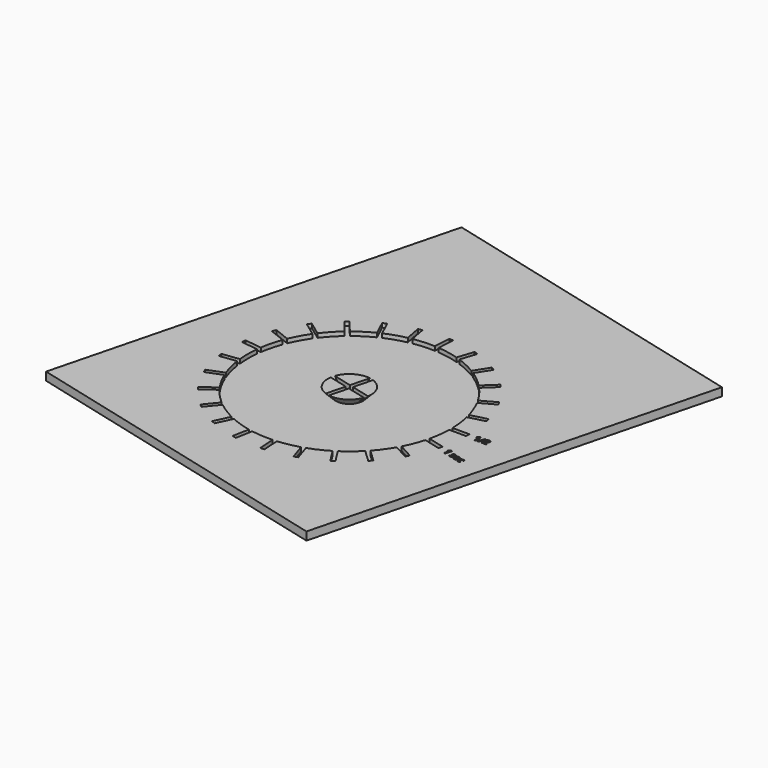
from build123d import *

# Parameters (mm, degrees)
F0_W          = 50
F0_H          = 60
F0_R          = 15
F2_DEPTH      = 0.6
F3_DEPTH      = 0.6
F4_R          = 2
F5_DEPTH      = 1.2
F5_TAPER      = -45
F6_W          = 0.6
F6_H          = 4.7
F6_H_2        = 0.6
F6_W_2        = 4.7
F7_DEPTH      = 0.8
F8_W          = 5
F8_H          = 0.6
F9_DEPTH      = 0.6
F10_TEXT_SIZE = 1.3888888889
F11_DEPTH     = 0.6
F12_ANGLE     = 14.4
F13_TEXT_SIZE = 1.3888888889
F14_DEPTH     = 0.6


# Not quite as in the source:
# - Text() gives the source's letters only with a copy of the font that has no kerning and outlines rounded to 1/6400 em; it was checked with that copy


with BuildPart() as f2:
    # F0 (on Top) → F2 (new body)
    with BuildSketch(Plane.XY):
        Rectangle(F0_W, F0_H)
        with Locations((0, -5)):
            Circle(F0_R, mode=Mode.SUBTRACT)
        with Locations((0, -5)):
            Circle(F0_R)
    extrude(amount=-F2_DEPTH)

    # F0 (on Top) → F3 (join)
    with BuildSketch(Plane.XY):
        Rectangle(F0_W, F0_H)
        with Locations((0, -5)):
            Circle(F0_R, mode=Mode.SUBTRACT)
    extrude(amount=F3_DEPTH)

    # F4 (on face) → F5 (join)
    with BuildSketch(Plane.XY):
        with Locations((0, -5)):
            Circle(F4_R)
    extrude(amount=F5_DEPTH, taper=F5_TAPER)

    # F6 (on face) → F7 (cut)
    with BuildSketch(Plane.XY.offset(1.2)):
        with Locations((0, -2.35)):
            Rectangle(F6_W, F6_H)
        with Locations((0, -5)):
            Rectangle(F6_W, F6_H_2)
        with Locations((-2.65, -5)):
            Rectangle(F6_W_2, F6_H_2)
        with Locations((2.65, -5)):
            Rectangle(F6_W_2, F6_H_2)
        with Locations((0, -7.65)):
            Rectangle(F6_W, F6_H)
    extrude(amount=-F7_DEPTH, mode=Mode.SUBTRACT)

    # F8 (on face) → F9 (cut)
    with BuildSketch(Plane.XY.offset(0.6)):
        with Locations((15, -5)):
            Rectangle(F8_W, F8_H)
        Polygon((17.0248122859, -0.938501923), (16.8755983536, -0.3573520263), (12.032682548, -1.6008014621), (12.1818964803, -2.1819513588), align=None)
        Polygon((15.479893003, 3.1677972928), (15.1908407985, 3.6935813008), (10.8093073983, 1.2848129303), (11.0983596028, 0.7590289223), align=None)
        Polygon((12.9623151117, 6.7608837655), (12.5515868481, 7.198264942), (8.906743711, 3.7755294123), (9.3174719745, 3.3381482359), align=None)
        Polygon((9.6302672898, 9.6149906578), (9.1236705345, 9.9364867348), (6.4445365596, 5.7148471073), (6.9511333149, 5.3933510303), align=None)
        Polygon((5.6931143565, 11.5507839369), (5.1224804467, 11.7361941335), (3.5773954748, 6.980911552), (4.1480293846, 6.7955013554), align=None)
        Polygon((1.3982421103, 12.4466305916), (0.7994260732, 12.4843049034), (0.4854734756, 7.4941712612), (1.0842895126, 7.4564969495), align=None)
        Polygon((-2.98448683, 12.2462412821), (-3.5738591805, 12.1338124934), (-2.6369526075, 7.2223762397), (-2.0475802571, 7.3348050285), align=None)
        Polygon((-7.1796894866, 10.9622072056), (-7.7225857181, 10.7067396307), (-5.5936892603, 6.1826043684), (-5.0507930288, 6.4380719433), align=None)
        Polygon((-10.9237658478, 8.6752089455), (-11.3860737934, 8.2927545517), (-8.1989538447, 4.4401883378), (-7.736645899, 4.8226427316), align=None)
        Polygon((-13.9814618259, 5.5289470134), (-14.3341329772, 5.0435368168), (-10.2890480054, 2.1046105553), (-9.936376854, 2.590020752), align=None)
        Polygon((-16.1606511372, 1.7211126177), (-16.3815258688, 1.1632467262), (-11.7326434394, -0.6773760372), (-11.5117687078, -0.1195101457), align=None)
        Polygon((-17.3244073029, -2.5090340022), (-17.3996072431, -3.104302823), (-12.4390337365, -3.7309689908), (-12.3638337964, -3.1357001701), align=None)
        Polygon((-17.3996072431, -6.895697177), (-17.3244073029, -7.4909659978), (-12.3638337964, -6.8642998299), (-12.4390337365, -6.2690310092), align=None)
        Polygon((-16.3815258688, -11.1632467262), (-16.1606511372, -11.7211126177), (-11.5117687078, -9.8804898543), (-11.7326434394, -9.3226239628), align=None)
        Polygon((-14.3341329772, -15.0435368168), (-13.9814618259, -15.5289470134), (-9.936376854, -12.590020752), (-10.2890480054, -12.1046105553), align=None)
        Polygon((-11.3860737934, -18.2927545517), (-10.9237658478, -18.6752089455), (-7.736645899, -14.8226427316), (-8.1989538447, -14.4401883378), align=None)
        Polygon((-7.7225857181, -20.7067396307), (-7.1796894866, -20.9622072056), (-5.0507930288, -16.4380719433), (-5.5936892603, -16.1826043684), align=None)
        Polygon((-3.5738591805, -22.1338124934), (-2.98448683, -22.2462412821), (-2.0475802571, -17.3348050285), (-2.6369526075, -17.2223762397), align=None)
        Polygon((0.7994260732, -22.4843049034), (1.3982421103, -22.4466305916), (1.0842895126, -17.4564969495), (0.4854734756, -17.4941712612), align=None)
        Polygon((5.1224804467, -21.7361941335), (5.6931143565, -21.5507839369), (4.1480293846, -16.7955013554), (3.5773954748, -16.980911552), align=None)
        Polygon((9.1236705345, -19.9364867348), (9.6302672898, -19.6149906578), (6.9511333149, -15.3933510303), (6.4445365596, -15.7148471073), align=None)
        Polygon((12.5515868481, -17.198264942), (12.9623151117, -16.7608837655), (9.3174719745, -13.3381482359), (8.906743711, -13.7755294123), align=None)
        Polygon((15.1908407985, -13.6935813008), (15.479893003, -13.1677972928), (11.0983596028, -10.7590289223), (10.8093073983, -11.2848129303), align=None)
        Polygon((16.8755983536, -9.6426479737), (17.0248122859, -9.061498077), (12.1818964803, -7.8180486412), (12.032682548, -8.3991985379), align=None)
    extrude(amount=-F9_DEPTH, mode=Mode.SUBTRACT)

    # F10 (on face) → F11 (cut, through all)
    with BuildSketch(Plane.XY.offset(0.6)):
        with Locations((18.5, -5.5)):
            Text('1 sec', F10_TEXT_SIZE, font='Open Sans', font_style=FontStyle.BOLD, text_align=(TextAlign.LEFT, TextAlign.BOTTOM))
    extrude(amount=-F11_DEPTH, mode=Mode.SUBTRACT)


with BuildPart() as f2_1:
    # F12: moved
    add(f2.part.rotate(Axis((0, -5, 4.7012548894), (0, 0, -1)), F12_ANGLE))

    # F13 (on face) → F14 (cut, through all)
    with BuildSketch(Plane.XY.offset(0.6)):
        with Locations((18.5, -5.5)):
            Text('1/2', F13_TEXT_SIZE, font='Open Sans', font_style=FontStyle.BOLD, text_align=(TextAlign.LEFT, TextAlign.BOTTOM))
    extrude(amount=-F14_DEPTH, mode=Mode.SUBTRACT)


solid = f2_1.part
